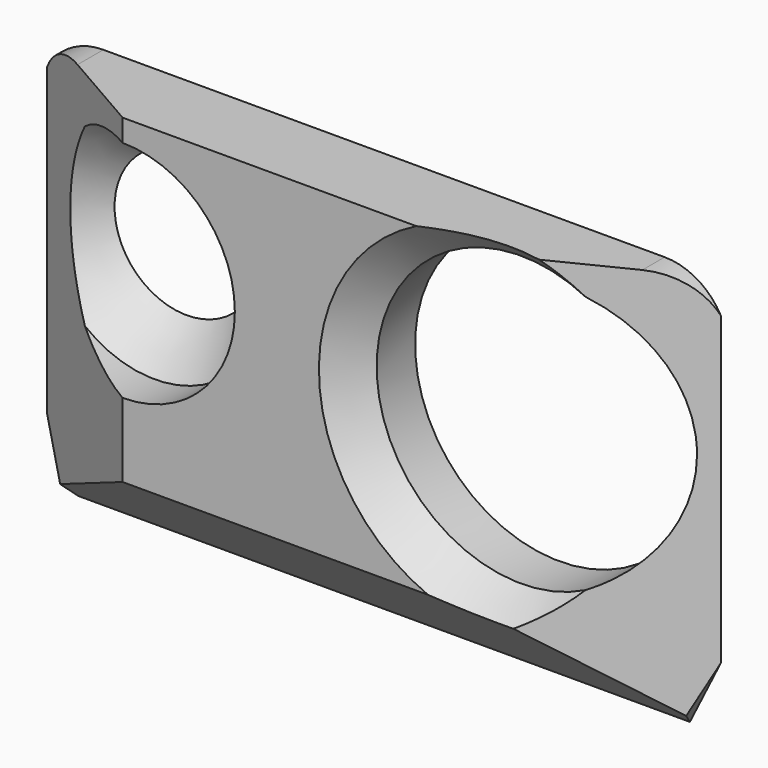
from build123d import *

# Parameters (mm, degrees)
F1_R        = 4.5
F1_R_2      = 9
F2_DEPTH    = 5
F3_R        = 7
F4_DEPTH    = 2
F6_S5_R     = 7
F6_T6_DEPTH = 12
F8_DEPTH    = 25.002
F11_REACH   = 49.0720678119


# Not quite as in the source:
# - a fillet or chamfer that OpenCascade refuses, or shapes differently, is made with other operations: its cross-section is extruded or revolved along the edge and cut away or added


with BuildPart() as f2:
    # F1 (on Front) → F2 (new body)
    with BuildSketch(Plane.XZ):
        with BuildLine():
            ThreePointArc((-17.5, 21.3840905163), (-19.5315060063, 20.829810085), (-21, 19.3205821894))
            Line((-21, 19.3205821894), (-21, 0.2360721162))
            Line((-21, 0.2360721162), (-19.0729714288, -3.6179094837))
            Line((-19.0729714288, -3.6179094837), (19.0729714288, -3.6179094837))
            Line((19.0729714288, -3.6179094837), (21, 0.2360721162))
            Line((21, 0.2360721162), (21, 19.3205821894))
            ThreePointArc((21, 19.3205821894), (19.5315060063, 20.829810085), (17.5, 21.3840905163))
            Line((17.5, 21.3840905163), (-17.5, 21.3840905163))
        make_face()
        with Locations((-12.3, 13)):
            Circle(F1_R, mode=Mode.SUBTRACT)
        with Locations((10.94, 11.55)):
            Circle(F1_R_2, mode=Mode.SUBTRACT)
    extrude(amount=F2_DEPTH)

    # F3 (on face) → F4 (cut)
    with BuildSketch(Plane.XZ.offset(5)):
        with Locations((-12.3, 13)):
            Circle(F3_R)
    extrude(amount=-F4_DEPTH, mode=Mode.SUBTRACT)

    # F5: chamfer of 2 on 1 edges, made by hand

    # F5_s1 → F5_t2 (revolve, cut)
    with BuildSketch(Plane.XY.offset(11.55)):
        Polygon((21.94, -5), (19.94, -3), (19.94, -5), align=None)
    revolve(axis=Axis((10.94, -5, 11.55), (0, -1, 0)), mode=Mode.SUBTRACT)

    # F6: chamfer of 3 on 1 edges, made by hand


with BuildPart() as f6_tool2:
    # F6_s3 → F6_t4 (revolve)
    with BuildSketch(Plane.XY.offset(13)):
        Polygon((-7.8, 0), (-4.8, -3), (-7.8, -3), align=None)
    revolve(axis=Axis((-12.3, -3, 13), (0, 1, 0)))

    # F6_s5 → F6_t6 (intersect, symmetric)
    with BuildSketch(Plane.XZ.offset(1.5)):
        with Locations((-12.3, 13)):
            Circle(F6_S5_R)
    extrude(amount=F6_T6_DEPTH, both=True, mode=Mode.INTERSECT)


with BuildPart() as f2_1:
    add(f2.part)

    # F6_t1: cut F6_tool2
    add(f6_tool2.part, mode=Mode.SUBTRACT)

    # F7 (on face) → F8 (cut, through all)
    with BuildSketch(Plane(origin=(0, 0, -3.6179094837), x_dir=(1, 0, 0), z_dir=(0, 0, -1))):
        Polygon((-21, 5), (-21, 0), (-12.3, 5), align=None)
        Polygon((21, 5), (10.94, 5), (21, 0), align=None)
    extrude(amount=-F8_DEPTH, mode=Mode.SUBTRACT)

    f11_end = Plane(origin=(-17.3406659547, -2.1030655433, 7.002775246), x_dir=(-0.867013944, 0.4982838759, 0), z_dir=(-0.4982838759, -0.867013944, 0))
    # F10 (on offset) → F11 (cut, up to a plane its end follows)
    with BuildSketch(Plane.YZ.offset(21)):
        Polygon((-5, -3.6179094837), (0, -3.6179094837), (-5, 1.3820905163), align=None)
    f11_long = extrude(amount=-F11_REACH, mode=Mode.PRIVATE)
    add(split(f11_long, bisect_by=f11_end, keep=Keep.BOTTOM, mode=Mode.PRIVATE), mode=Mode.SUBTRACT)


solid = f2_1.part
